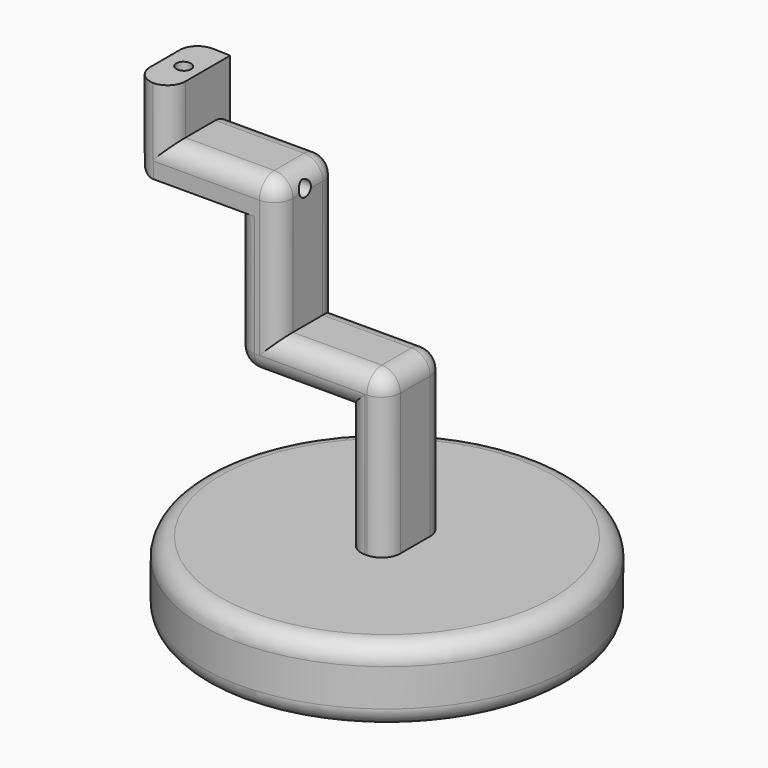
from build123d import *

# Parameters (mm, degrees)
F1_DEPTH       = 20
F2_R           = 49.5669200912
F3_DEPTH       = 20
F5_D           = 4
F5_DEPTH       = 20
F5_TIP         = 1.2017212381
F7_D           = 4
F9_D           = 10
F9_DEPTH       = 60.2140555616
F10_T1_DEPTH   = 41.3520902395
F10_T3_DEPTH   = 25.797053054
F10_T9_DEPTH   = 53.8520902395
F10_T13_DEPTH  = 38.297053054
F11_T1_DEPTH   = 47.8307861835
F12_S2_W       = 5.1
F12_S2_H       = 5.1
F12_T3_DEPTH   = 5.1
F12_S7_W       = 5.1
F12_S7_H       = 5.1
F12_T8_DEPTH   = 5.1
F12_S12_W      = 5.1
F12_S12_H      = 5.1
F12_T13_DEPTH  = 5.1
F12_S17_W      = 5.1
F12_S17_H      = 5.1
F12_T18_DEPTH  = 5.1
F12_S22_W      = 5.1
F12_S22_H      = 5.1
F12_T23_DEPTH  = 5.1
F12_S27_W      = 5.1
F12_S27_H      = 5.1
F12_T28_DEPTH  = 5.1
F12_T36_ANGLE  = 190.4069282709
F12_T39_ANGLE  = 187.8158071603
F12_T42_DEPTH  = 30.3307861835
F12_T45_DEPTH  = 22.0958729088
F12_T48_DEPTH  = 32.3822730035
F12_T51_DEPTH  = 24.604753945
F12_T54_DEPTH  = 32.8662917018
F12_T57_DEPTH  = 37.9018014111
F12_T60_DEPTH  = 23.8520907052
F12_T63_DEPTH  = 31.629609298
F12_T66_DEPTH  = 23.8520902395
F12_T69_DEPTH  = 10
F12_T72_DEPTH  = 37.9018014111
F12_T75_DEPTH  = 31.6296092979
F12_T78_DEPTH  = 23.8520907052
F12_T81_DEPTH  = 32.8662917018
F12_T84_DEPTH  = 24.604753945
F12_T87_DEPTH  = 32.3822730035
F12_T90_DEPTH  = 22.5
F12_T93_DEPTH  = 10
F12_T96_DEPTH  = 10
F12_T99_ANGLE  = 90.0000000014
F12_T103_DEPTH = 34.5958729088
F12_T108_DEPTH = 44.8822730035
F12_T115_DEPTH = 37.104753945
F12_T120_DEPTH = 45.3662917018
F12_T127_DEPTH = 36.3520907052
F12_T132_DEPTH = 44.129609298
F12_T139_DEPTH = 44.1296092979
F12_T144_DEPTH = 36.3520907052
F12_T151_DEPTH = 45.3662917018
F12_T156_DEPTH = 37.104753945


# Not quite as in the source:
# - a fillet or chamfer that OpenCascade refuses, or shapes differently, is made with other operations: its cross-section is extruded or revolved along the edge and cut away or added
# - two fillets or chamfers of one size are made in one step


with BuildPart() as f1:
    # F0 (on Front) → F1 (new body)
    with BuildSketch(Plane.XZ):
        Polygon((-50.6793223321, 43.4035807848), (-60.2130554616, 43.6544679105), (-60.2130554616, 20.8236817271), (-33.1171825528, 20.8236817271), (-33.1171825528, -16.5585912764), (-3.5124286078, -16.5585912764), (-3.5124286078, -49.4248829782), (7.0248586126, -49.4248829782), (7.0248586126, -6.5230815671), (-21.8272320926, -6.5230815671), (-21.8272320926, 30.1065277308), (-50.6793223321, 30.1065277308), align=None)
    extrude(amount=F1_DEPTH)

    # F2 (on face) → F3 (join)
    with BuildSketch(Plane(origin=(0, 0, -49.4248829782), x_dir=(1, 0, 0), z_dir=(0, 0, -1))):
        with Locations((0, 10.7094217092)):
            Circle(F2_R)
    extrude(amount=F3_DEPTH)

    # F5
    with Locations(Plane(origin=(1.1063343415, 0, 42.040803541), x_dir=(0.999653921, 0, -0.0263066205), z_dir=(0.0263066205, 0, 0.999653921))):
        with Locations((-56.2409870327, -10.0355511531)):
            Hole(F5_D / 2, depth=F5_DEPTH)
            with Locations((0, 0, -(F5_DEPTH + F5_TIP / 2))):  # 118° drill point
                Cone(0, F5_D / 2, F5_TIP, mode=Mode.SUBTRACT)

    # F7 (through all)
    with Locations(Plane.YZ.offset(-21.8272320926)):
        with Locations((-10.9037412331, 25.7294327021)):
            Hole(F7_D / 2)

    # F9 (through all, one way)
    with BuildSketch(Plane.YZ):
        with Locations((-9.5938993618, -67.5340369344)):
            Circle(F9_D / 2)
    extrude(amount=-F9_DEPTH, mode=Mode.SUBTRACT)

    # F10: fillet of radius 5 on 2 edges, made by hand

    # F10_s2 → F10_t1 (cut)
    with BuildSketch(Plane.YZ.offset(-50.6793223321)):
        with BuildLine():
            ThreePointArc((-15, 30.1065277308), (-18.5355339059, 28.6420616368), (-20, 25.1065277308))
            Line((-20, 25.1065277308), (-20, 30.1065277308))
            Line((-20, 30.1065277308), (-15, 30.1065277308))
        make_face()
    extrude(amount=F10_T1_DEPTH, mode=Mode.SUBTRACT)

    # F10_s4 → F10_t3 (cut)
    with BuildSketch(Plane.XY.offset(30.1065277308)):
        with BuildLine():
            ThreePointArc((-50.6793223321, -15), (-52.1437884262, -18.5355339059), (-55.6793223321, -20))
            Line((-55.6793223321, -20), (-50.6793223321, -20))
            Line((-50.6793223321, -20), (-50.6793223321, -15))
        make_face()
    extrude(amount=F10_T3_DEPTH, mode=Mode.SUBTRACT)


with BuildPart() as f10_tool7:
    # F10_s8 → F10_t9 (new body)
    with BuildSketch(Plane.YZ.offset(-9.3272320926)):
        with BuildLine():
            ThreePointArc((-15, 30.1065277308), (-18.5355339059, 28.6420616368), (-20, 25.1065277308))
            Line((-20, 25.1065277308), (-20, 30.1065277308))
            Line((-20, 30.1065277308), (-15, 30.1065277308))
        make_face()
    extrude(amount=-F10_T9_DEPTH)

    split(bisect_by=Plane.YZ.offset(-50.6793223321), keep=Keep.BOTTOM)


with BuildPart() as f10_tool11:
    # F10_s12 → F10_t13 (new body)
    with BuildSketch(Plane.XY.offset(17.6065277308)):
        with BuildLine():
            ThreePointArc((-50.6793223321, -15), (-52.1437884262, -18.5355339059), (-55.6793223321, -20))
            Line((-55.6793223321, -20), (-50.6793223321, -20))
            Line((-50.6793223321, -20), (-50.6793223321, -15))
        make_face()
    extrude(amount=F10_T13_DEPTH)

    split(bisect_by=Plane.XY.offset(30.1065277308), keep=Keep.BOTTOM)


with BuildPart() as f10_tool7_1:
    add(f10_tool7.part)

    # F10_t15: intersect F10_tool11
    add(f10_tool11.part, mode=Mode.INTERSECT)


with BuildPart() as f1_1:
    add(f1.part)

    # F10_t5: cut F10_tool7
    add(f10_tool7_1.part, mode=Mode.SUBTRACT)

    # F11: fillet of radius 5 on 1 edges, made by hand

    # F11_s2 → F11_t1 (cut)
    with BuildSketch(Plane.XY.offset(8.3236817271)):
        with BuildLine():
            ThreePointArc((-60.2130554616, -15), (-58.7485893676, -18.5355339059), (-55.2130554616, -20))
            Line((-55.2130554616, -20), (-60.2130554616, -20))
            Line((-60.2130554616, -20), (-60.2130554616, -15))
        make_face()
    extrude(amount=F11_T1_DEPTH, mode=Mode.SUBTRACT)

    # F12: fillet of radius 5 on 23 edges, made by hand


with BuildPart() as f12_tool1:
    # F12_s2 → F12_t3 (new body)
    with BuildSketch(Plane.YZ.offset(-55.2130554616)):
        with Locations((-2.45, 23.2736817271)):
            Rectangle(F12_S2_W, F12_S2_H)
    extrude(amount=-F12_T3_DEPTH)

    # F12_s4 → F12_t5 (revolve, cut)
    with BuildSketch(Plane(origin=(-55.2130554616, -5, 25.8236817271), x_dir=(0, -0.7071067812, 0.7071067812), z_dir=(0, -0.7071067812, -0.7071067812))):
        with BuildLine():
            ThreePointArc((0, -5), (5, 0), (0, 5))
            Line((0, 5), (0, -5))
        make_face()
    revolve(axis=Axis((-55.2130554616, -5, 25.8236817271), (-1, 0, 0)), mode=Mode.SUBTRACT)


with BuildPart() as f12_tool6:
    # F12_s7 → F12_t8 (new body)
    with BuildSketch(Plane.XY.offset(-11.5585912764)):
        with Locations((-30.6671825528, -2.45)):
            Rectangle(F12_S7_W, F12_S7_H)
    extrude(amount=-F12_T8_DEPTH)

    # F12_s9 → F12_t10 (revolve, cut)
    with BuildSketch(Plane(origin=(-28.1171825528, -5, -11.5585912764), x_dir=(0.7071067812, -0.7071067812, 0), z_dir=(0.7071067812, 0.7071067812, 0))):
        with BuildLine():
            ThreePointArc((0, -5), (5, 0), (0, 5))
            Line((0, 5), (0, -5))
        make_face()
    revolve(axis=Axis((-28.1171825528, -5, -11.5585912764), (0, 0, -1)), mode=Mode.SUBTRACT)


with BuildPart() as f12_tool11:
    # F12_s12 → F12_t13 (new body)
    with BuildSketch(Plane.XZ.offset(5)):
        with Locations((4.5748586126, -8.9730815671)):
            Rectangle(F12_S12_W, F12_S12_H)
    extrude(amount=-F12_T13_DEPTH)

    # F12_s14 → F12_t15 (revolve, cut)
    with BuildSketch(Plane(origin=(2.0248586126, -5, -11.5230815671), x_dir=(-0.7071067812, 0, -0.7071067812), z_dir=(0.7071067812, 0, -0.7071067812))):
        with BuildLine():
            ThreePointArc((0, -5), (5, 0), (0, 5))
            Line((0, 5), (0, -5))
        make_face()
    revolve(axis=Axis((2.0248586126, -5, -11.5230815671), (0, 1, 0)), mode=Mode.SUBTRACT)


with BuildPart() as f12_tool16:
    # F12_s17 → F12_t18 (new body)
    with BuildSketch(Plane.XY.offset(25.1065277308)):
        with Locations((-24.2772320926, -2.45)):
            Rectangle(F12_S17_W, F12_S17_H)
    extrude(amount=F12_T18_DEPTH)

    # F12_s19 → F12_t20 (revolve, cut)
    with BuildSketch(Plane(origin=(-26.8272320926, -5, 25.1065277308), x_dir=(-0.7071067812, -0.7071067812, 0), z_dir=(-0.7071067812, 0.7071067812, 0))):
        with BuildLine():
            ThreePointArc((0, -5), (5, 0), (0, 5))
            Line((0, 5), (0, -5))
        make_face()
    revolve(axis=Axis((-26.8272320926, -5, 25.1065277308), (0, 0, 1)), mode=Mode.SUBTRACT)


with BuildPart() as f12_tool21:
    # F12_s22 → F12_t23 (new body)
    with BuildSketch(Plane.YZ.offset(2.0248586126)):
        with Locations((-17.55, -8.9730815671)):
            Rectangle(F12_S22_W, F12_S22_H)
    extrude(amount=F12_T23_DEPTH)

    # F12_s24 → F12_t25 (revolve, cut)
    with BuildSketch(Plane(origin=(2.0248586126, -15, -11.5230815671), x_dir=(0, 0.7071067812, -0.7071067812), z_dir=(0, -0.7071067812, -0.7071067812))):
        with BuildLine():
            ThreePointArc((0, -5), (5, 0), (0, 5))
            Line((0, 5), (0, -5))
        make_face()
    revolve(axis=Axis((2.0248586126, -15, -11.5230815671), (1, 0, 0)), mode=Mode.SUBTRACT)


with BuildPart() as f12_tool26:
    # F12_s27 → F12_t28 (new body)
    with BuildSketch(Plane.YZ.offset(-28.1171825528)):
        with Locations((-17.55, -14.1085912764)):
            Rectangle(F12_S27_W, F12_S27_H)
    extrude(amount=-F12_T28_DEPTH)

    # F12_s29 → F12_t30 (revolve, cut)
    with BuildSketch(Plane(origin=(-28.1171825528, -15, -11.5585912764), x_dir=(0, 0.7071067812, 0.7071067812), z_dir=(0, -0.7071067812, 0.7071067812))):
        with BuildLine():
            ThreePointArc((0, -5), (5, 0), (0, 5))
            Line((0, 5), (0, -5))
        make_face()
    revolve(axis=Axis((-28.1171825528, -15, -11.5585912764), (-1, 0, 0)), mode=Mode.SUBTRACT)


with BuildPart() as f12_tool31:
    # F12_s32 → F12_t33 (revolve)
    with BuildSketch(Plane.XZ.offset(10.7094217092)):
        with BuildLine():
            ThreePointArc((49.5669200912, -54.4248829782), (48.1024539971, -50.8893490723), (44.5669200912, -49.4248829782))
            Line((44.5669200912, -49.4248829782), (49.5669200912, -49.4248829782))
            Line((49.5669200912, -49.4248829782), (49.5669200912, -54.4248829782))
        make_face()
    revolve(axis=Axis((0, -10.7094217092, -49.4248829782), (0, 0, -1)))


with BuildPart() as f12_tool34:
    # F12_s35 → F12_t36 (revolve)
    with BuildSketch(Plane.XZ.offset(10.7094217092)):
        with BuildLine():
            ThreePointArc((49.5669200912, -64.4248829782), (48.1024539971, -67.9604168841), (44.5669200912, -69.4248829782))
            Line((44.5669200912, -69.4248829782), (49.5669200912, -69.4248829782))
            Line((49.5669200912, -69.4248829782), (49.5669200912, -64.4248829782))
        make_face()
    revolve(axis=Axis((0, -10.7094217092, -69.4248829782), (0, 0, -1)), revolution_arc=F12_T36_ANGLE)


with BuildPart() as f12_tool37:
    # F12_s38 → F12_t39 (revolve)
    with BuildSketch(Plane(origin=(1.4428334137, -10.5113725728, 0), x_dir=(0, 0, 1), z_dir=(0.1359889017, -0.9907103606, 0))):
        with BuildLine():
            ThreePointArc((-64.4248829782, 51.0232825873), (-67.9604168841, 49.5588164933), (-69.4248829782, 46.0232825873))
            Line((-69.4248829782, 46.0232825873), (-69.4248829782, 51.0232825873))
            Line((-69.4248829782, 51.0232825873), (-64.4248829782, 51.0232825873))
        make_face()
    revolve(axis=Axis((0, -10.7094217092, -69.4248829782), (0, 0, -1)), revolution_arc=F12_T39_ANGLE)


with BuildPart() as f12_tool40:
    # F12_s41 → F12_t42 (new body)
    with BuildSketch(Plane.XY.offset(56.1544679105)):
        with BuildLine():
            ThreePointArc((-55.2130554616, 0), (-58.7485893676, -1.4644660941), (-60.2130554616, -5))
            Line((-60.2130554616, -5), (-60.2130554616, 0))
            Line((-60.2130554616, 0), (-55.2130554616, 0))
        make_face()
    extrude(amount=-F12_T42_DEPTH)


with BuildPart() as f12_tool43:
    # F12_s44 → F12_t45 (new body)
    with BuildSketch(Plane.YZ.offset(-55.2130554616)):
        with BuildLine():
            ThreePointArc((0, 25.8236817271), (-1.4644660941, 22.2881478211), (-5, 20.8236817271))
            Line((-5, 20.8236817271), (0, 20.8236817271))
            Line((0, 20.8236817271), (0, 25.8236817271))
        make_face()
    extrude(amount=F12_T45_DEPTH)


with BuildPart() as f12_tool46:
    # F12_s47 → F12_t48 (new body)
    with BuildSketch(Plane.XY.offset(20.8236817271)):
        with BuildLine():
            ThreePointArc((-28.1171825528, 0), (-31.6527164587, -1.4644660941), (-33.1171825528, -5))
            Line((-33.1171825528, -5), (-33.1171825528, 0))
            Line((-33.1171825528, 0), (-28.1171825528, 0))
        make_face()
    extrude(amount=-F12_T48_DEPTH)


with BuildPart() as f12_tool49:
    # F12_s50 → F12_t51 (new body)
    with BuildSketch(Plane.YZ.offset(-28.1171825528)):
        with BuildLine():
            ThreePointArc((0, -11.5585912764), (-1.4644660941, -15.0941251823), (-5, -16.5585912764))
            Line((-5, -16.5585912764), (0, -16.5585912764))
            Line((0, -16.5585912764), (0, -11.5585912764))
        make_face()
    extrude(amount=F12_T51_DEPTH)


with BuildPart() as f12_tool52:
    # F12_s53 → F12_t54 (new body)
    with BuildSketch(Plane.XY.offset(-16.5585912764)):
        with BuildLine():
            ThreePointArc((1.4875713922, 0), (-2.0479625137, -1.4644660941), (-3.5124286078, -5))
            Line((-3.5124286078, -5), (-3.5124286078, 0))
            Line((-3.5124286078, 0), (1.4875713922, 0))
        make_face()
    extrude(amount=-F12_T54_DEPTH)


with BuildPart() as f12_tool55:
    # F12_s56 → F12_t57 (new body)
    with BuildSketch(Plane.XY.offset(-49.4248829782)):
        with BuildLine():
            ThreePointArc((2.0248586126, 0), (5.5603925185, -1.4644660941), (7.0248586126, -5))
            Line((7.0248586126, -5), (7.0248586126, 0))
            Line((7.0248586126, 0), (2.0248586126, 0))
        make_face()
    extrude(amount=F12_T57_DEPTH)


with BuildPart() as f12_tool58:
    # F12_s59 → F12_t60 (new body)
    with BuildSketch(Plane.YZ.offset(2.0248586126)):
        with BuildLine():
            ThreePointArc((0, -11.5230815671), (-1.4644660941, -7.9875476612), (-5, -6.5230815671))
            Line((-5, -6.5230815671), (0, -6.5230815671))
            Line((0, -6.5230815671), (0, -11.5230815671))
        make_face()
    extrude(amount=-F12_T60_DEPTH)


with BuildPart() as f12_tool61:
    # F12_s62 → F12_t63 (new body)
    with BuildSketch(Plane.XY.offset(-6.5230815671)):
        with BuildLine():
            ThreePointArc((-26.8272320926, 0), (-23.2916981867, -1.4644660941), (-21.8272320926, -5))
            Line((-21.8272320926, -5), (-21.8272320926, 0))
            Line((-21.8272320926, 0), (-26.8272320926, 0))
        make_face()
    extrude(amount=F12_T63_DEPTH)


with BuildPart() as f12_tool64:
    # F12_s65 → F12_t66 (new body)
    with BuildSketch(Plane.YZ.offset(-26.8272320926)):
        with BuildLine():
            ThreePointArc((0, 25.1065277308), (-1.4644660941, 28.6420616368), (-5, 30.1065277308))
            Line((-5, 30.1065277308), (0, 30.1065277308))
            Line((0, 30.1065277308), (0, 25.1065277308))
        make_face()
    extrude(amount=-F12_T66_DEPTH)


with BuildPart() as f12_tool67:
    # F12_s68 → F12_t69 (new body)
    with BuildSketch(Plane.XZ.offset(5)):
        with BuildLine():
            ThreePointArc((7.0248586126, -11.5230815671), (5.5603925185, -7.9875476612), (2.0248586126, -6.5230815671))
            Line((2.0248586126, -6.5230815671), (7.0248586126, -6.5230815671))
            Line((7.0248586126, -6.5230815671), (7.0248586126, -11.5230815671))
        make_face()
    extrude(amount=F12_T69_DEPTH)


with BuildPart() as f12_tool70:
    # F12_s71 → F12_t72 (new body)
    with BuildSketch(Plane.XY.offset(-49.4248829782)):
        with BuildLine():
            ThreePointArc((7.0248586126, -15), (5.5603925185, -18.5355339059), (2.0248586126, -20))
            Line((2.0248586126, -20), (7.0248586126, -20))
            Line((7.0248586126, -20), (7.0248586126, -15))
        make_face()
    extrude(amount=F12_T72_DEPTH)


with BuildPart() as f12_tool73:
    # F12_s74 → F12_t75 (new body)
    with BuildSketch(Plane.XY.offset(-6.5230815671)):
        with BuildLine():
            ThreePointArc((-26.8272320926, -20), (-23.2916981867, -18.5355339059), (-21.8272320926, -15))
            Line((-21.8272320926, -15), (-21.8272320926, -20))
            Line((-21.8272320926, -20), (-26.8272320926, -20))
        make_face()
    extrude(amount=F12_T75_DEPTH)


with BuildPart() as f12_tool76:
    # F12_s77 → F12_t78 (new body)
    with BuildSketch(Plane.YZ.offset(2.0248586126)):
        with BuildLine():
            ThreePointArc((-20, -11.5230815671), (-18.5355339059, -7.9875476612), (-15, -6.5230815671))
            Line((-15, -6.5230815671), (-20, -6.5230815671))
            Line((-20, -6.5230815671), (-20, -11.5230815671))
        make_face()
    extrude(amount=-F12_T78_DEPTH)


with BuildPart() as f12_tool79:
    # F12_s80 → F12_t81 (new body)
    with BuildSketch(Plane.XY.offset(-16.5585912764)):
        with BuildLine():
            ThreePointArc((1.4875713922, -20), (-2.0479625137, -18.5355339059), (-3.5124286078, -15))
            Line((-3.5124286078, -15), (-3.5124286078, -20))
            Line((-3.5124286078, -20), (1.4875713922, -20))
        make_face()
    extrude(amount=-F12_T81_DEPTH)


with BuildPart() as f12_tool82:
    # F12_s83 → F12_t84 (new body)
    with BuildSketch(Plane.YZ.offset(-28.1171825528)):
        with BuildLine():
            ThreePointArc((-20, -11.5585912764), (-18.5355339059, -15.0941251823), (-15, -16.5585912764))
            Line((-15, -16.5585912764), (-20, -16.5585912764))
            Line((-20, -16.5585912764), (-20, -11.5585912764))
        make_face()
    extrude(amount=F12_T84_DEPTH)


with BuildPart() as f12_tool85:
    # F12_s86 → F12_t87 (new body)
    with BuildSketch(Plane.XY.offset(20.8236817271)):
        with BuildLine():
            ThreePointArc((-28.1171825528, -20), (-31.6527164587, -18.5355339059), (-33.1171825528, -15))
            Line((-33.1171825528, -15), (-33.1171825528, -20))
            Line((-33.1171825528, -20), (-28.1171825528, -20))
        make_face()
    extrude(amount=-F12_T87_DEPTH)


with BuildPart() as f12_tool88:
    # F12_s89 → F12_t90 (new body)
    with BuildSketch(Plane.XZ.offset(5)):
        with BuildLine():
            ThreePointArc((-60.2130554616, 25.8236817271), (-58.7485893676, 22.2881478211), (-55.2130554616, 20.8236817271))
            Line((-55.2130554616, 20.8236817271), (-60.2130554616, 20.8236817271))
            Line((-60.2130554616, 20.8236817271), (-60.2130554616, 25.8236817271))
        make_face()
    extrude(amount=F12_T90_DEPTH)


with BuildPart() as f12_tool91:
    # F12_s92 → F12_t93 (new body)
    with BuildSketch(Plane.XZ.offset(5)):
        with BuildLine():
            ThreePointArc((-33.1171825528, -11.5585912764), (-31.6527164587, -15.0941251823), (-28.1171825528, -16.5585912764))
            Line((-28.1171825528, -16.5585912764), (-33.1171825528, -16.5585912764))
            Line((-33.1171825528, -16.5585912764), (-33.1171825528, -11.5585912764))
        make_face()
    extrude(amount=F12_T93_DEPTH)


with BuildPart() as f12_tool94:
    # F12_s95 → F12_t96 (new body)
    with BuildSketch(Plane.XZ.offset(5)):
        with BuildLine():
            ThreePointArc((-21.8272320926, 25.1065277308), (-23.2916981867, 28.6420616368), (-26.8272320926, 30.1065277308))
            Line((-26.8272320926, 30.1065277308), (-21.8272320926, 30.1065277308))
            Line((-21.8272320926, 30.1065277308), (-21.8272320926, 25.1065277308))
        make_face()
    extrude(amount=F12_T96_DEPTH)


with BuildPart() as f12_tool97:
    # F12_s98 → F12_t99 (revolve)
    with BuildSketch(Plane.XY.offset(25.1065277309)):
        with BuildLine():
            ThreePointArc((-21.8272320926, -15), (-23.2916981867, -18.5355339059), (-26.8272320926, -20))
            Line((-26.8272320926, -20), (-21.8272320926, -20))
            Line((-21.8272320926, -20), (-21.8272320926, -15))
        make_face()
    revolve(axis=Axis((-21.8272320926, -15.0000000001, 25.1065277309), (-1, 0, 0)), revolution_arc=F12_T99_ANGLE)


with BuildPart() as f12_tool101:
    # F12_s102 → F12_t103 (new body)
    with BuildSketch(Plane.YZ.offset(-55.2130554616)):
        with BuildLine():
            ThreePointArc((0, 25.8236817271), (-1.4644660941, 22.2881478211), (-5, 20.8236817271))
            Line((-5, 20.8236817271), (0, 20.8236817271))
            Line((0, 20.8236817271), (0, 25.8236817271))
        make_face()
    extrude(amount=F12_T103_DEPTH)

    split(bisect_by=Plane.YZ.offset(-33.1171825528), keep=Keep.TOP)

    split(bisect_by=Plane.YZ.offset(-21.8272320926), keep=Keep.BOTTOM)


with BuildPart() as f12_tool106:
    # F12_s107 → F12_t108 (new body)
    with BuildSketch(Plane.XY.offset(33.3236817271)):
        with BuildLine():
            ThreePointArc((-28.1171825528, 0), (-31.6527164587, -1.4644660941), (-33.1171825528, -5))
            Line((-33.1171825528, -5), (-33.1171825528, 0))
            Line((-33.1171825528, 0), (-28.1171825528, 0))
        make_face()
    extrude(amount=-F12_T108_DEPTH)

    split(bisect_by=Plane.XY.offset(20.8236817271), keep=Keep.TOP)

    split(bisect_by=Plane.XY.offset(30.1065277308), keep=Keep.BOTTOM)


with BuildPart() as f12_tool101_1:
    add(f12_tool101.part)

    # F12_t111: intersect F12_tool106
    add(f12_tool106.part, mode=Mode.INTERSECT)


with BuildPart() as f12_tool113:
    # F12_s114 → F12_t115 (new body)
    with BuildSketch(Plane.YZ.offset(-28.1171825528)):
        with BuildLine():
            ThreePointArc((0, -11.5585912764), (-1.4644660941, -15.0941251823), (-5, -16.5585912764))
            Line((-5, -16.5585912764), (0, -16.5585912764))
            Line((0, -16.5585912764), (0, -11.5585912764))
        make_face()
    extrude(amount=F12_T115_DEPTH)

    split(bisect_by=Plane.YZ.offset(7.0248586126), keep=Keep.BOTTOM)

    split(bisect_by=Plane.YZ.offset(-3.5124286078), keep=Keep.TOP)


with BuildPart() as f12_tool118:
    # F12_s119 → F12_t120 (new body)
    with BuildSketch(Plane.XY.offset(-4.0585912764)):
        with BuildLine():
            ThreePointArc((1.4875713922, 0), (-2.0479625137, -1.4644660941), (-3.5124286078, -5))
            Line((-3.5124286078, -5), (-3.5124286078, 0))
            Line((-3.5124286078, 0), (1.4875713922, 0))
        make_face()
    extrude(amount=-F12_T120_DEPTH)

    split(bisect_by=Plane.XY.offset(-16.5585912764), keep=Keep.TOP)

    split(bisect_by=Plane.XY.offset(-6.5230815671), keep=Keep.BOTTOM)


with BuildPart() as f12_tool113_1:
    add(f12_tool113.part)

    # F12_t123: intersect F12_tool118
    add(f12_tool118.part, mode=Mode.INTERSECT)


with BuildPart() as f12_tool125:
    # F12_s126 → F12_t127 (new body)
    with BuildSketch(Plane.YZ.offset(2.0248586126)):
        with BuildLine():
            ThreePointArc((0, -11.5230815671), (-1.4644660941, -7.9875476612), (-5, -6.5230815671))
            Line((-5, -6.5230815671), (0, -6.5230815671))
            Line((0, -6.5230815671), (0, -11.5230815671))
        make_face()
    extrude(amount=-F12_T127_DEPTH)

    split(bisect_by=Plane.YZ.offset(-33.1171825528), keep=Keep.TOP)

    split(bisect_by=Plane.YZ.offset(-21.8272320926), keep=Keep.BOTTOM)


with BuildPart() as f12_tool130:
    # F12_s131 → F12_t132 (new body)
    with BuildSketch(Plane.XY.offset(-19.0230815671)):
        with BuildLine():
            ThreePointArc((-26.8272320926, 0), (-23.2916981867, -1.4644660941), (-21.8272320926, -5))
            Line((-21.8272320926, -5), (-21.8272320926, 0))
            Line((-21.8272320926, 0), (-26.8272320926, 0))
        make_face()
    extrude(amount=F12_T132_DEPTH)

    split(bisect_by=Plane.XY.offset(-16.5585912764), keep=Keep.TOP)

    split(bisect_by=Plane.XY.offset(-6.5230815671), keep=Keep.BOTTOM)


with BuildPart() as f12_tool125_1:
    add(f12_tool125.part)

    # F12_t135: intersect F12_tool130
    add(f12_tool130.part, mode=Mode.INTERSECT)


with BuildPart() as f12_tool137:
    # F12_s138 → F12_t139 (new body)
    with BuildSketch(Plane.XY.offset(-19.0230815671)):
        with BuildLine():
            ThreePointArc((-26.8272320926, -20), (-23.2916981867, -18.5355339059), (-21.8272320926, -15))
            Line((-21.8272320926, -15), (-21.8272320926, -20))
            Line((-21.8272320926, -20), (-26.8272320926, -20))
        make_face()
    extrude(amount=F12_T139_DEPTH)

    split(bisect_by=Plane.XY.offset(-16.5585912764), keep=Keep.TOP)

    split(bisect_by=Plane.XY.offset(-6.5230815671), keep=Keep.BOTTOM)


with BuildPart() as f12_tool142:
    # F12_s143 → F12_t144 (new body)
    with BuildSketch(Plane.YZ.offset(2.0248586126)):
        with BuildLine():
            ThreePointArc((-20, -11.5230815671), (-18.5355339059, -7.9875476612), (-15, -6.5230815671))
            Line((-15, -6.5230815671), (-20, -6.5230815671))
            Line((-20, -6.5230815671), (-20, -11.5230815671))
        make_face()
    extrude(amount=-F12_T144_DEPTH)

    split(bisect_by=Plane.YZ.offset(-33.1171825528), keep=Keep.TOP)

    split(bisect_by=Plane.YZ.offset(-21.8272320926), keep=Keep.BOTTOM)


with BuildPart() as f12_tool137_1:
    add(f12_tool137.part)

    # F12_t147: intersect F12_tool142
    add(f12_tool142.part, mode=Mode.INTERSECT)


with BuildPart() as f12_tool149:
    # F12_s150 → F12_t151 (new body)
    with BuildSketch(Plane.XY.offset(-4.0585912764)):
        with BuildLine():
            ThreePointArc((1.4875713922, -20), (-2.0479625137, -18.5355339059), (-3.5124286078, -15))
            Line((-3.5124286078, -15), (-3.5124286078, -20))
            Line((-3.5124286078, -20), (1.4875713922, -20))
        make_face()
    extrude(amount=-F12_T151_DEPTH)

    split(bisect_by=Plane.XY.offset(-16.5585912764), keep=Keep.TOP)

    split(bisect_by=Plane.XY.offset(-6.5230815671), keep=Keep.BOTTOM)


with BuildPart() as f12_tool154:
    # F12_s155 → F12_t156 (new body)
    with BuildSketch(Plane.YZ.offset(-28.1171825528)):
        with BuildLine():
            ThreePointArc((-20, -11.5585912764), (-18.5355339059, -15.0941251823), (-15, -16.5585912764))
            Line((-15, -16.5585912764), (-20, -16.5585912764))
            Line((-20, -16.5585912764), (-20, -11.5585912764))
        make_face()
    extrude(amount=F12_T156_DEPTH)

    split(bisect_by=Plane.YZ.offset(7.0248586126), keep=Keep.BOTTOM)

    split(bisect_by=Plane.YZ.offset(-3.5124286078), keep=Keep.TOP)


with BuildPart() as f12_tool149_1:
    add(f12_tool149.part)

    # F12_t159: intersect F12_tool154
    add(f12_tool154.part, mode=Mode.INTERSECT)


with BuildPart() as f1_2:
    add(f1_1.part)

    # F12_t160: cut F12_tool1, F12_tool6, F12_tool11, F12_tool16, F12_tool21, F12_tool26, F12_tool31, F12_tool34, F12_tool37, F12_tool40, F12_tool43, F12_tool46, F12_tool49, F12_tool52, F12_tool55, F12_tool58, F12_tool61, F12_tool64, F12_tool67, F12_tool70, F12_tool73, F12_tool76, F12_tool79, F12_tool82, F12_tool85, F12_tool88, F12_tool91, F12_tool94, F12_tool97, F12_tool101, F12_tool113, F12_tool125, F12_tool137, F12_tool149
    add([f12_tool1.part, f12_tool6.part, f12_tool11.part, f12_tool16.part, f12_tool21.part, f12_tool26.part, f12_tool31.part, f12_tool34.part, f12_tool37.part, f12_tool40.part, f12_tool43.part, f12_tool46.part, f12_tool49.part, f12_tool52.part, f12_tool55.part, f12_tool58.part, f12_tool61.part, f12_tool64.part, f12_tool67.part, f12_tool70.part, f12_tool73.part, f12_tool76.part, f12_tool79.part, f12_tool82.part, f12_tool85.part, f12_tool88.part, f12_tool91.part, f12_tool94.part, f12_tool97.part, f12_tool101_1.part, f12_tool113_1.part, f12_tool125_1.part, f12_tool137_1.part, f12_tool149_1.part], mode=Mode.SUBTRACT)


solid = f1_2.part
